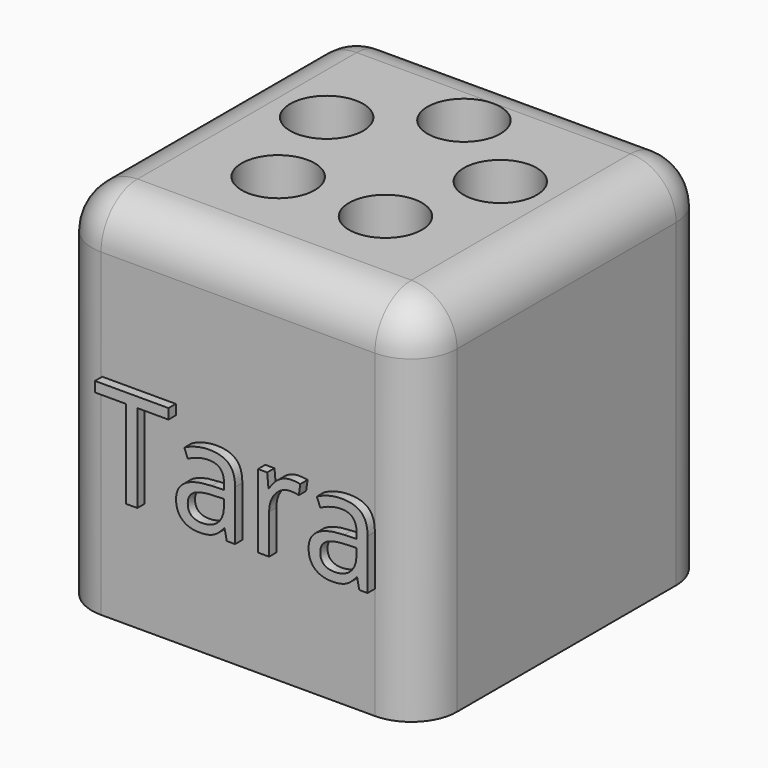
from build123d import *

# Parameters (mm, degrees)
F0_W         = 40
F0_H         = 40
F1_DEPTH     = 20
F3_R         = 5
F2_R         = 4
F4_DEPTH     = 35
F5_TEXT_SIZE = 15.0541006743
F6_DEPTH     = 1


# Not quite as in the source:
# - Text() gives the source's letters only with a copy of the font that has no kerning and outlines rounded to 1/6400 em; it was checked with that copy


with BuildPart() as f1:
    # F0 (on Right) → F1 (new body, symmetric)
    with BuildSketch(Plane.YZ):
        with Locations((-0.9450220622, 20)):
            Rectangle(F0_W, F0_H)
    extrude(amount=F1_DEPTH, both=True)

    # F3
    f3_edges = [f1.edges().sort_by_distance(p)[0] for p in [
        (20, -20.945022, 20),
        (20, 19.054978, 20),
        (-20, 19.054978, 20),
        (-20, -20.945022, 20),
        (0, -20.945022, 40),
        (20, -0.945022, 40),
        (0, 19.054978, 40),
        (-20, -0.945022, 40),
    ]]
    fillet(f3_edges, radius=F3_R)

    # F2 (on face) → F4 (cut)
    with BuildSketch(Plane.XY.offset(40)):
        with Locations((0, 10)):
            Circle(F2_R)
        with Locations((-9.510565163, 3.0901699437)):
            Circle(F2_R)
        with Locations((-5.8778525229, -8.0901699437)):
            Circle(F2_R)
        with Locations((5.8778525229, -8.0901699437)):
            Circle(F2_R)
        with Locations((9.510565163, 3.0901699437)):
            Circle(F2_R)
    extrude(amount=-F4_DEPTH, mode=Mode.SUBTRACT)

    # F5 (on face) → F6 (join)
    with BuildSketch(Plane.XZ.offset(20.9450220622)):
        with Locations((-15, 12.2674484389)):
            Text('Tara', F5_TEXT_SIZE, font='Open Sans', text_align=(TextAlign.LEFT, TextAlign.BOTTOM))
    extrude(amount=F6_DEPTH)


solid = f1.part
